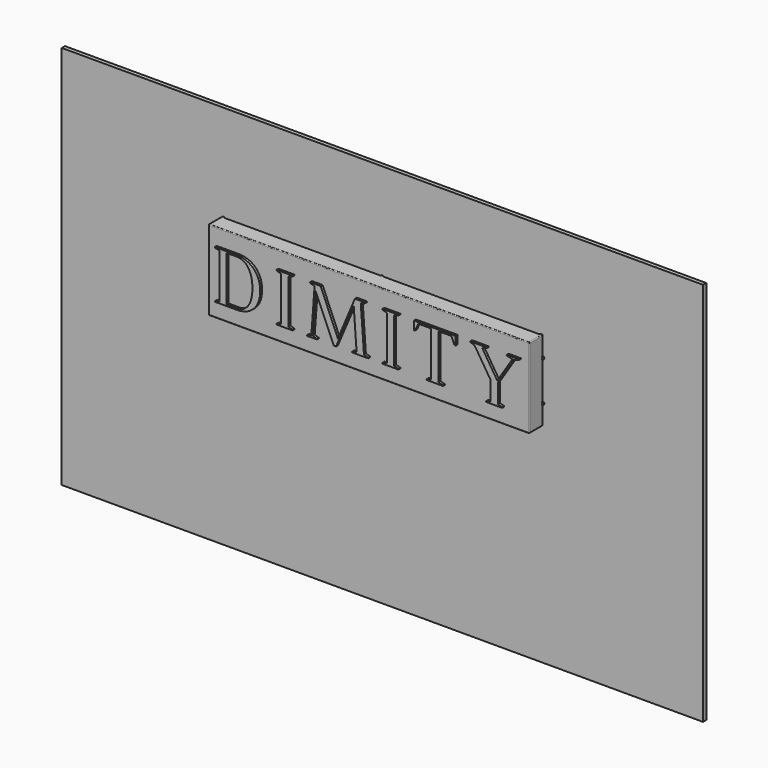
from build123d import *

# Parameters (mm, degrees)
F1_DEPTH          = 15
F2_W              = 2000
F2_H              = 500
F3_DEPTH          = 100
F5_DEPTH          = 6
F4_W              = 20
F4_H              = 500
F7_D              = 4.3
F7_DEPTH          = 12
F7_CBORE_D        = 7.5
F7_CBORE_DEPTH    = 2
F7_TIP            = 1.2918503309
F7_2_D            = 4.3
F7_2_DEPTH        = 12
F7_2_CBORE_D      = 7.5
F7_2_CBORE_DEPTH  = 2
F7_2_TIP          = 1.2918503309
F9_D              = 4.3
F9_DEPTH          = 12
F9_CBORE_D        = 7.5
F9_CBORE_DEPTH    = 2
F9_TIP            = 1.2918503309
F9_2_D            = 4.3
F9_2_DEPTH        = 12
F9_2_CBORE_D      = 7.5
F9_2_CBORE_DEPTH  = 2
F9_2_TIP          = 1.2918503309
F11_D             = 4.3
F11_DEPTH         = 12
F11_CBORE_D       = 7.5
F11_CBORE_DEPTH   = 2
F11_TIP           = 1.2918503309
F11_2_D           = 4.3
F11_2_DEPTH       = 12
F11_2_CBORE_D     = 7.5
F11_2_CBORE_DEPTH = 2
F11_2_TIP         = 1.2918503309
F12_R             = 5
F13_R             = 5
F13_2_R           = 5
F14_R             = 5
F15_D             = 4.3
F15_DEPTH         = 12
F15_CBORE_D       = 7.5
F15_CBORE_DEPTH   = 2
F15_TIP           = 1.2918503309
F17_D             = 4.3
F17_DEPTH         = 12
F17_CBORE_D       = 7.5
F17_CBORE_DEPTH   = 2
F17_TIP           = 1.2918503309
F19_D             = 4.3
F19_DEPTH         = 12
F19_CBORE_D       = 7.5
F19_CBORE_DEPTH   = 2
F19_TIP           = 1.2918503309
F20_R             = 5
F21_W             = 1000
F21_H             = 2400
F22_DEPTH         = 25


# Not quite as in the source:
# - a feature names something its author has since deleted; it is built from what else it names


with BuildPart() as f1:
    # F0 (on Front) → F1 (new body)
    with BuildSketch(Plane.XZ):
        with BuildLine():
            Line((-811.4863290109, 190.8960236935), (-948.4822653052, 190.8960236935))
            Line((-948.4822653052, 190.8960236935), (-948.4822653052, 187.026470246))
            Line((-948.4822653052, 187.026470246), (-920.5675615954, 180.5855808972))
            Line((-920.5675615954, 180.5855808972), (-920.5675615954, -99.4144191028))
            Line((-920.5675615954, -99.4144191028), (-948.4822653052, -106.2880248782))
            Line((-948.4822653052, -106.2880248782), (-948.4822653052, -109.7185700347))
            Line((-948.4822653052, -109.7185700347), (-811.4863290109, -109.7185700347))
            add(Edge.make_bspline(
                [(-811.4863290109, -109.7185700347), (-725.5950765146, -109.7185700347), (-665.4719211129, -53.8951927924), (-665.4719211129, 40.5855808972)],
                knots=[0, 0, 0, 0, 1, 1, 1, 1], degree=3))
            add(Edge.make_bspline(
                [(-665.4719211129, 40.5855808972), (-665.4719211129, 134.2074070186), (-725.5950765146, 190.8960236935), (-811.4863290109, 190.8960236935)],
                knots=[0, 0, 0, 0, 1, 1, 1, 1], degree=3))
        make_face()
        with BuildLine():
            Line((-874.1893877168, -101.1328034801), (-874.1893877168, 182.3039994076))
            Line((-874.1893877168, 182.3039994076), (-811.4863290109, 182.3039994076))
            add(Edge.make_bspline(
                [(-811.4863290109, 182.3039994076), (-754.7954481751, 182.3039994076), (-714.0012413063, 135.0653647276), (-714.0012413063, 40.1591222018)],
                knots=[0, 0, 0, 0, 1, 1, 1, 1], degree=3))
            add(Edge.make_bspline(
                [(-714.0012413063, 40.1591222018), (-714.0012413063, -54.3216514878), (-754.7954481751, -101.1328034801), (-811.4863290109, -101.1328034801)],
                knots=[0, 0, 0, 0, 1, 1, 1, 1], degree=3))
            Line((-811.4863290109, -101.1328034801), (-874.1893877168, -101.1328034801))
        make_face(mode=Mode.SUBTRACT)
    extrude(amount=F1_DEPTH)


with BuildPart() as f1b:
    # F0 (on Front) → F1, piece 2 (new body)
    with BuildSketch(Plane.XZ):
        Polygon((-463.1765365311, 190.8960236935), (-563.2455211101, 190.8960236935), (-563.2455211101, 186.6000115506), (-535.3245482914, 178.4407036914), (-535.3245482914, -97.2695418969), (-563.2455211101, -105.428815623), (-563.2455211101, -109.7185700347), (-463.1765365311, -109.7185700347), (-463.1765365311, -105.428815623), (-489.8055495349, -97.2695418969), (-489.8055495349, 178.4407036914), (-463.1765365311, 186.6000115506), align=None)
    extrude(amount=F1_DEPTH)


with BuildPart() as f1c:
    # F0 (on Front) → F1, piece 3 (new body)
    with BuildSketch(Plane.XZ):
        Polygon((-288.3881929127, 190.8960236935), (-354.0953039465, 190.8960236935), (-354.0953039465, 186.6000115506), (-326.1806002367, 178.4407036914), (-346.3687466471, -98.1287511521), (-374.2771926257, -106.2880248782), (-374.2771926257, -109.7185700347), (-311.1476752244, -109.7185700347), (-311.1476752244, -106.2880248782), (-337.3502522882, -98.1287511521), (-318.8805243881, 151.8179484188), (-206.7952394757, -109.7185700347), (-192.6214895855, -109.7185700347), (-82.2546231834, 151.3851978591), (-64.2113539788, -97.2695418969), (-92.1323154199, -105.428815623), (-92.1323154199, -109.7185700347), (8.3631164769, -109.7185700347), (8.3631164769, -105.428815623), (-18.2659306599, -97.2695418969), (-38.0150574017, 178.4407036914), (-11.3922793737, 186.6000115506), (-11.3922793737, 190.8960236935), (-74.5217967751, 190.8960236935), (-181.0254129717, -62.4811869009), align=None)
    extrude(amount=F1_DEPTH)


with BuildPart() as f1d:
    # F0 (on Front) → F1, piece 4 (new body)
    with BuildSketch(Plane.XZ):
        Polygon((196.4847853017, 190.8960236935), (96.4220698316, 190.8960236935), (96.4220698316, 186.6000115506), (124.3367735414, 178.4407036914), (124.3367735414, -97.2695418969), (96.4220698316, -105.428815623), (96.4220698316, -109.7185700347), (196.4847853017, -109.7185700347), (196.4847853017, -105.428815623), (169.8620414068, -97.2695418969), (169.8620414068, 178.4407036914), (196.4847853017, 186.6000115506), align=None)
    extrude(amount=F1_DEPTH)


with BuildPart() as f1e:
    # F0 (on Front) → F1, piece 5 (new body)
    with BuildSketch(Plane.XZ):
        Polygon((554.2270267512, 190.8960236935), (293.5497061751, 190.8960236935), (293.5497061751, 138.0707027349), (300.4170542193, 138.0707027349), (320.6052006298, 182.3039994076), (400.4797696895, 182.3039994076), (400.4797696895, -97.2695418969), (372.5650659796, -105.428815623), (372.5650659796, -109.7185700347), (474.7789163869, -109.7185700347), (474.7789163869, -105.428815623), (446.864212677, -97.2695418969), (446.864212677, 182.3039994076), (527.1777900278, 182.3039994076), (546.9269281472, 138.0707027349), (554.2270267512, 138.0707027349), align=None)
    extrude(amount=F1_DEPTH)


with BuildPart() as f1f:
    # F0 (on Front) → F1, piece 6 (new body)
    with BuildSketch(Plane.XZ):
        Polygon((747.9303756695, 190.8960236935), (644.4308231785, 190.8960236935), (644.4308231785, 186.6000115506), (671.0536012065, 178.4407036914), (771.549044481, 20.8301850466), (771.549044481, -97.2695418969), (743.6343635266, -105.428815623), (743.6343635266, -109.7185700347), (844.1235376921, -109.7185700347), (844.1235376921, -105.428815623), (817.5007596642, -97.2695418969), (817.5007596642, 20.8301850466), (917.9899338298, 178.4407036914), (948.4822653052, 186.6000115506), (948.4822653052, 190.8960236935), (872.0445105109, 190.8960236935), (872.0445105109, 186.6000115506), (908.1184879468, 178.4407036914), (813.2110052525, 30.2814185876), (719.5891791311, 178.4407036914), (747.9303756695, 186.6000115506), align=None)
    extrude(amount=F1_DEPTH)


with BuildPart() as f3:
    # F2 (on Front) → F3 (new body)
    with BuildSketch(Plane.XZ):
        with Locations((0, 43.4922596839)):
            Rectangle(F2_W, F2_H)
    extrude(amount=-F3_DEPTH)

    # F7
    with Locations(Plane(origin=(0, 106, 0), x_dir=(-1, 0, 0), z_dir=(0, 1, 0))):
        with Locations((-990, 268.4922596839), (-990, 43.4922596839), (-990, -181.5077403161)):
            CounterBoreHole(F7_D / 2, F7_CBORE_D / 2, F7_CBORE_DEPTH, depth=F7_DEPTH)
            with Locations((0, 0, -(F7_DEPTH + F7_TIP / 2))):  # 118° drill point
                Cone(0, F7_D / 2, F7_TIP, mode=Mode.SUBTRACT)

    # F9
    with Locations(Plane(origin=(0, 106, 0), x_dir=(-1, 0, 0), z_dir=(0, 1, 0))):
        with Locations((0, 268.4922596839), (0, -181.5077403161), (0, 43.4922596839)):
            CounterBoreHole(F9_D / 2, F9_CBORE_D / 2, F9_CBORE_DEPTH, depth=F9_DEPTH)
            with Locations((0, 0, -(F9_DEPTH + F9_TIP / 2))):  # 118° drill point
                Cone(0, F9_D / 2, F9_TIP, mode=Mode.SUBTRACT)

    # F11
    with Locations(Plane(origin=(0, 106, 0), x_dir=(-1, 0, 0), z_dir=(0, 1, 0))):
        with Locations((990, 268.4922596839), (990, -181.5077403161)):
            CounterBoreHole(F11_D / 2, F11_CBORE_D / 2, F11_CBORE_DEPTH, depth=F11_DEPTH)
            with Locations((0, 0, -(F11_DEPTH + F11_TIP / 2))):  # 118° drill point
                Cone(0, F11_D / 2, F11_TIP, mode=Mode.SUBTRACT)

    # F12
    f12_edges = [f3.edges().sort_by_distance(p)[0] for p in [
        (1000, 50, 293.49226),
        (1000, 50, -206.50774),
        (-1000, 50, 293.49226),
        (-1000, 50, -206.50774),
    ]]
    fillet(f12_edges, radius=F12_R)

    # F20
    f20_edges = [f3.edges().sort_by_distance(p)[0] for p in [
        (-1000, 0, 43.49226),
        (0, 0, 293.49226),
    ]]
    fillet(f20_edges, radius=F20_R)


with BuildPart() as f5:
    # F4 (on face) → F5 (new body)
    with BuildSketch(Plane(origin=(0, 100, 0), x_dir=(-1, 0, 0), z_dir=(0, 1, 0))):
        with BuildLine():
            Line((-1000, -91.5077403161), (-1000, -206.5077403161))
            Line((-1000, -206.5077403161), (-980, -206.5077403161))
            Line((-980, -206.5077403161), (-980, 293.4922596839))
            Line((-980, 293.4922596839), (-1000, 293.4922596839))
            Line((-1000, 293.4922596839), (-1000, 178.4922596839))
            ThreePointArc((-1000, 178.4922596839), (-992.9289321881, 175.5633274957), (-990, 168.4922596839))
            ThreePointArc((-990, 168.4922596839), (-992.9289321881, 161.421191872), (-1000, 158.4922596839))
            Line((-1000, 158.4922596839), (-1000, -71.5077403161))
            ThreePointArc((-1000, -71.5077403161), (-992.9289321881, -74.4366725043), (-990, -81.5077403161))
            ThreePointArc((-990, -81.5077403161), (-992.9289321881, -88.578808128), (-1000, -91.5077403161))
        make_face()
        with BuildLine():
            ThreePointArc((-1000, -71.5077403161), (-1010, -81.5077403161), (-1000, -91.5077403161))
            Line((-1000, -91.5077403161), (-1000, -71.5077403161))
        make_face()
        with BuildLine():
            Line((-1000, -71.5077403161), (-1000, -91.5077403161))
            ThreePointArc((-1000, -91.5077403161), (-992.9289321881, -88.578808128), (-990, -81.5077403161))
            ThreePointArc((-990, -81.5077403161), (-992.9289321881, -74.4366725043), (-1000, -71.5077403161))
        make_face()
        with BuildLine():
            ThreePointArc((-1000, 178.4922596839), (-1010, 168.4922596839), (-1000, 158.4922596839))
            Line((-1000, 158.4922596839), (-1000, 178.4922596839))
        make_face()
        with BuildLine():
            Line((-1000, 178.4922596839), (-1000, 158.4922596839))
            ThreePointArc((-1000, 158.4922596839), (-992.9289321881, 161.421191872), (-990, 168.4922596839))
            ThreePointArc((-990, 168.4922596839), (-992.9289321881, 175.5633274957), (-1000, 178.4922596839))
        make_face()
    extrude(amount=F5_DEPTH)

    # F7#2
    with Locations(Plane(origin=(0, 106, 0), x_dir=(-1, 0, 0), z_dir=(0, 1, 0))):
        with Locations((-990, 268.4922596839), (-990, 43.4922596839), (-990, -181.5077403161)):
            CounterBoreHole(F7_2_D / 2, F7_2_CBORE_D / 2, F7_2_CBORE_DEPTH, depth=F7_2_DEPTH)
            with Locations((0, 0, -(F7_2_DEPTH + F7_2_TIP / 2))):  # 118° drill point
                Cone(0, F7_2_D / 2, F7_2_TIP, mode=Mode.SUBTRACT)

    # F13#2
    f13_2_edges = [f5.edges().sort_by_distance(p)[0] for p in [
        (980, 103, -206.50774),
        (1000, 103, -206.50774),
        (1000, 103, 293.49226),
        (980, 103, 293.49226),
    ]]
    fillet(f13_2_edges, radius=F13_2_R)

    # F19
    with Locations(Plane.XZ.offset(-100)):
        with Locations((1005, 168.492259681), (1005.0331354141, -81.5077403161)):
            CounterBoreHole(F19_D / 2, F19_CBORE_D / 2, F19_CBORE_DEPTH, depth=F19_DEPTH)
            with Locations((0, 0, -(F19_DEPTH + F19_TIP / 2))):  # 118° drill point
                Cone(0, F19_D / 2, F19_TIP, mode=Mode.SUBTRACT)


with BuildPart() as f5b:
    # F4 (on face) → F5, piece 2 (new body)
    with BuildSketch(Plane(origin=(0, 100, 0), x_dir=(-1, 0, 0), z_dir=(0, 1, 0))):
        with Locations((0, 43.4922596839)):
            Rectangle(F4_W, F4_H)
    extrude(amount=F5_DEPTH)

    # F9#2
    with Locations(Plane(origin=(0, 106, 0), x_dir=(-1, 0, 0), z_dir=(0, 1, 0))):
        with Locations((0, 268.4922596839), (0, -181.5077403161), (0, 43.4922596839)):
            CounterBoreHole(F9_2_D / 2, F9_2_CBORE_D / 2, F9_2_CBORE_DEPTH, depth=F9_2_DEPTH)
            with Locations((0, 0, -(F9_2_DEPTH + F9_2_TIP / 2))):  # 118° drill point
                Cone(0, F9_2_D / 2, F9_2_TIP, mode=Mode.SUBTRACT)

    # F14
    f14_edges = [f5b.edges().sort_by_distance(p)[0] for p in [
        (10, 103, 293.49226),
        (-10, 103, 293.49226),
        (-10, 103, -206.50774),
        (10, 103, -206.50774),
    ]]
    fillet(f14_edges, radius=F14_R)

    # F15
    with Locations(Plane(origin=(0, 100, 0), x_dir=(-1, 0, 0), z_dir=(0, -1, 0))):
        with Locations((0, -168.4922596839), (0, 81.5077403161)):
            CounterBoreHole(F15_D / 2, F15_CBORE_D / 2, F15_CBORE_DEPTH, depth=F15_DEPTH)
            with Locations((0, 0, -(F15_DEPTH + F15_TIP / 2))):  # 118° drill point
                Cone(0, F15_D / 2, F15_TIP, mode=Mode.SUBTRACT)


with BuildPart() as f5c:
    # F4 (on face) → F5, piece 3 (new body)
    with BuildSketch(Plane(origin=(0, 100, 0), x_dir=(-1, 0, 0), z_dir=(0, 1, 0))):
        with BuildLine():
            Line((980, -206.5077403161), (1000, -206.5077403161))
            Line((1000, -206.5077403161), (1000, -91.5077403161))
            ThreePointArc((1000, -91.5077403161), (990, -81.5077403161), (1000, -71.5077403161))
            Line((1000, -71.5077403161), (1000, 158.4922596839))
            ThreePointArc((1000, 158.4922596839), (990, 168.4922596839), (1000, 178.4922596839))
            Line((1000, 178.4922596839), (1000, 293.4922596839))
            Line((1000, 293.4922596839), (980, 293.4922596839))
            Line((980, 293.4922596839), (980, -206.5077403161))
        make_face()
        with BuildLine():
            ThreePointArc((1000, -71.5077403161), (990, -81.5077403161), (1000, -91.5077403161))
            Line((1000, -91.5077403161), (1000, -71.5077403161))
        make_face()
        with BuildLine():
            Line((1000, -71.5077403161), (1000, -91.5077403161))
            ThreePointArc((1000, -91.5077403161), (1007.0710678119, -88.578808128), (1010, -81.5077403161))
            ThreePointArc((1010, -81.5077403161), (1007.0710678119, -74.4366725043), (1000, -71.5077403161))
        make_face()
        with BuildLine():
            ThreePointArc((1000, 178.4922596839), (990, 168.4922596839), (1000, 158.4922596839))
            Line((1000, 158.4922596839), (1000, 178.4922596839))
        make_face()
        with BuildLine():
            Line((1000, 178.4922596839), (1000, 158.4922596839))
            ThreePointArc((1000, 158.4922596839), (1007.0710678119, 161.421191872), (1010, 168.4922596839))
            ThreePointArc((1010, 168.4922596839), (1007.0710678119, 175.5633274957), (1000, 178.4922596839))
        make_face()
    extrude(amount=F5_DEPTH)

    # F11#2
    with Locations(Plane(origin=(0, 106, 0), x_dir=(-1, 0, 0), z_dir=(0, 1, 0))):
        with Locations((990, 268.4922596839), (990, -181.5077403161)):
            CounterBoreHole(F11_2_D / 2, F11_2_CBORE_D / 2, F11_2_CBORE_DEPTH, depth=F11_2_DEPTH)
            with Locations((0, 0, -(F11_2_DEPTH + F11_2_TIP / 2))):  # 118° drill point
                Cone(0, F11_2_D / 2, F11_2_TIP, mode=Mode.SUBTRACT)

    # F13
    f13_edges = [f5c.edges().sort_by_distance(p)[0] for p in [
        (-1000, 103, 293.49226),
        (-980, 103, 293.49226),
        (-980, 103, -206.50774),
        (-1000, 103, -206.50774),
    ]]
    fillet(f13_edges, radius=F13_R)

    # F17
    with Locations(Plane.XZ.offset(-100)):
        with Locations((-1005, 168.4922596839), (-1005, -81.5077403161)):
            CounterBoreHole(F17_D / 2, F17_CBORE_D / 2, F17_CBORE_DEPTH, depth=F17_DEPTH)
            with Locations((0, 0, -(F17_DEPTH + F17_TIP / 2))):  # 118° drill point
                Cone(0, F17_D / 2, F17_TIP, mode=Mode.SUBTRACT)


with BuildPart() as f22:
    # F21 (on face) → F22 (new body)
    with BuildSketch(Plane(origin=(0, 106, 0), x_dir=(-1, 0, 0), z_dir=(0, 1, 0))):
        with Locations((-500, -307.2351396084)):
            Rectangle(F21_W, F21_H)
        with Locations((500, -307.2351396084)):
            Rectangle(F21_W, F21_H)
        with Locations((-1500, -307.2351396084)):
            Rectangle(F21_W, F21_H)
        with Locations((1500, -307.2351396084)):
            Rectangle(F21_W, F21_H)
    extrude(amount=F22_DEPTH)


solid = Compound([f1.part, f1b.part, f1c.part, f1d.part, f1e.part, f1f.part, f3.part, f5.part, f5b.part, f5c.part, f22.part])
